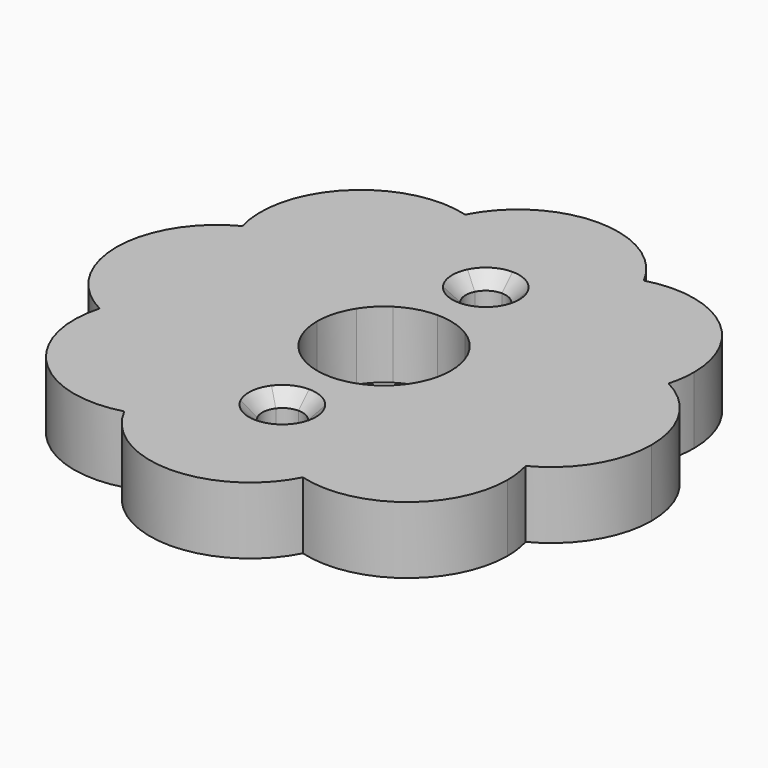
from build123d import *

# Parameters (mm, degrees)
F1_DEPTH = 6.35
F2_SIZE  = 1.27


with BuildPart() as f1:
    # F0 (on Top) → F1 (new body)
    with BuildSketch(Plane.XY):
        with BuildLine():
            Line((9.0862708935, 13.0175), (13.0175, 9.0862708935))
            ThreePointArc((13.0175, 9.0862708935), (11.2253201513, 11.2253201513), (9.0862708935, 13.0175))
        make_face()
        with BuildLine():
            ThreePointArc((20.221779693, 8.4753248493), (16.6798616454, 9.4909337123), (13.0175, 9.0862708935))
            ThreePointArc((13.0175, 9.0862708935), (14.680846164, 6.0405613073), (15.6426389263, 2.7061914978))
            ThreePointArc((15.6426389263, 2.7061914978), (18.5124203716, 5.1302265884), (20.221779693, 8.4753248493))
        make_face()
        with BuildLine():
            ThreePointArc((9.0862708935, 13.0175), (11.2253201513, 11.2253201513), (13.0175, 9.0862708935))
            ThreePointArc((13.0175, 9.0862708935), (16.6798616454, 9.4909337123), (20.221779693, 8.4753248493))
            ThreePointArc((20.221779693, 8.4753248493), (20.4876913926, 9.751427392), (20.5768854467, 11.0518854467))
            ThreePointArc((20.5768854467, 11.0518854467), (16.8044451078, 18.6435705262), (8.4753248493, 20.221779693))
            ThreePointArc((8.4753248493, 20.221779693), (9.2588631643, 18.1108617814), (9.525, 15.875))
            ThreePointArc((9.525, 15.875), (9.4146788384, 14.4295079143), (9.0862708935, 13.0175))
        make_face()
        with BuildLine():
            ThreePointArc((15.6426389263, 2.7061914978), (14.680846164, 6.0405613073), (13.0175, 9.0862708935))
            ThreePointArc((13.0175, 9.0862708935), (9.0369714008, 6.6307608822), (6.7051057537, 2.5765605975))
            ThreePointArc((6.7051057537, 2.5765605975), (11.1900224972, 1.5278871711), (15.6426389263, 2.7061914978))
        make_face()
        with BuildLine():
            ThreePointArc((6.7051057537, 2.5765605975), (9.0369714008, 6.6307608822), (13.0175, 9.0862708935))
            Line((13.0175, 9.0862708935), (9.0862708935, 13.0175))
            ThreePointArc((9.0862708935, 13.0175), (6.6307608822, 9.0369714008), (2.5765605975, 6.7051057537))
            ThreePointArc((2.5765605975, 6.7051057537), (2.9714834378, 6.0087982599), (3.4234793231, 5.3481108183))
            ThreePointArc((3.4234793231, 5.3481108183), (4.4901280605, 4.4901280605), (5.3481108183, 3.4234793231))
            ThreePointArc((5.3481108183, 3.4234793231), (6.0087982599, 2.9714834378), (6.7051057537, 2.5765605975))
        make_face()
        with BuildLine():
            ThreePointArc((2.5765605975, 6.7051057537), (6.6307608822, 9.0369714008), (9.0862708935, 13.0175))
            ThreePointArc((9.0862708935, 13.0175), (6.0405613073, 14.680846164), (2.7061914978, 15.6426389263))
            ThreePointArc((2.7061914978, 15.6426389263), (2.1024733841, 14.3128130347), (1.7091513138, 12.9063244241))
            ThreePointArc((1.7091513138, 12.9063244241), (1.8553919064, 12.4969095665), (1.905, 12.065))
            ThreePointArc((1.905, 12.065), (1.8082177094, 11.465522131), (1.5277047607, 10.9269564313))
            ThreePointArc((1.5277047607, 10.9269564313), (1.8078843831, 8.7553512461), (2.5765605975, 6.7051057537))
        make_face()
        with BuildLine():
            ThreePointArc((2.7061914978, 15.6426389263), (6.0405613073, 14.680846164), (9.0862708935, 13.0175))
            ThreePointArc((9.0862708935, 13.0175), (9.4146788384, 14.4295079143), (9.525, 15.875))
            ThreePointArc((9.525, 15.875), (9.2588631643, 18.1108617814), (8.4753248493, 20.221779693))
            ThreePointArc((8.4753248493, 20.221779693), (5.1302265884, 18.5124203716), (2.7061914978, 15.6426389263))
        make_face()
        with BuildLine():
            ThreePointArc((20.221779693, 8.4753248493), (18.5124203716, 5.1302265884), (15.6426389263, 2.7061914978))
            ThreePointArc((15.6426389263, 2.7061914978), (15.8168030581, 1.3580743804), (15.875, 0))
            ThreePointArc((15.875, 0), (15.8168030581, -1.3580743804), (15.6426389263, -2.7061914978))
            ThreePointArc((15.6426389263, -2.7061914978), (18.5124203716, -5.1302265884), (20.221779693, -8.4753248493))
            ThreePointArc((20.221779693, -8.4753248493), (24.0029979569, -4.9660119021), (25.4, 0))
            ThreePointArc((25.4, 0), (24.0029979569, 4.9660119021), (20.221779693, 8.4753248493))
        make_face()
        with BuildLine():
            ThreePointArc((15.875, 0), (15.8168030581, 1.3580743804), (15.6426389263, 2.7061914978))
            ThreePointArc((15.6426389263, 2.7061914978), (11.1900224972, 1.5278871711), (6.7051057537, 2.5765605975))
            ThreePointArc((6.7051057537, 2.5765605975), (6.4391940541, 1.3004580548), (6.35, 0))
            Line((6.35, 0), (15.875, 0))
        make_face()
        with BuildLine():
            ThreePointArc((6.35, 0), (6.4391940541, 1.3004580548), (6.7051057537, 2.5765605975))
            ThreePointArc((6.7051057537, 2.5765605975), (6.0087982599, 2.9714834378), (5.3481108183, 3.4234793231))
            ThreePointArc((5.3481108183, 3.4234793231), (6.0943828111, 1.783535296), (6.35, 0))
        make_face()
        with BuildLine():
            ThreePointArc((1.7091513138, 12.9063244241), (2.1024733841, 14.3128130347), (2.7061914978, 15.6426389263))
            ThreePointArc((2.7061914978, 15.6426389263), (1.3580743804, 15.8168030581), (0, 15.875))
            Line((0, 15.875), (0, 13.97))
            ThreePointArc((0, 13.97), (1.0065540155, 13.6823663821), (1.7091513138, 12.9063244241))
        make_face()
        with BuildLine():
            ThreePointArc((0, 15.875), (1.3580743804, 15.8168030581), (2.7061914978, 15.6426389263))
            ThreePointArc((2.7061914978, 15.6426389263), (5.1302265884, 18.5124203716), (8.4753248493, 20.221779693))
            ThreePointArc((8.4753248493, 20.221779693), (0, 25.4), (-8.4753248493, 20.221779693))
            ThreePointArc((-8.4753248493, 20.221779693), (-5.1302265884, 18.5124203716), (-2.7061914978, 15.6426389263))
            ThreePointArc((-2.7061914978, 15.6426389263), (-1.3580743804, 15.8168030581), (0, 15.875))
        make_face()
        with BuildLine():
            ThreePointArc((3.4234793231, 5.3481108183), (2.9714834378, 6.0087982599), (2.5765605975, 6.7051057537))
            ThreePointArc((2.5765605975, 6.7051057537), (1.3004580548, 6.4391940541), (0, 6.35))
            ThreePointArc((0, 6.35), (1.783535296, 6.0943828111), (3.4234793231, 5.3481108183))
        make_face()
        with BuildLine():
            ThreePointArc((0, 6.35), (1.3004580548, 6.4391940541), (2.5765605975, 6.7051057537))
            ThreePointArc((2.5765605975, 6.7051057537), (1.8078843831, 8.7553512461), (1.5277047607, 10.9269564313))
            ThreePointArc((1.5277047607, 10.9269564313), (0.8547081378, 10.3625021295), (0, 10.16))
            Line((0, 10.16), (0, 6.35))
        make_face()
        with BuildLine():
            ThreePointArc((15.6426389263, -2.7061914978), (15.8168030581, -1.3580743804), (15.875, 0))
            Line((15.875, 0), (6.35, 0))
            ThreePointArc((6.35, 0), (6.4391940541, -1.3004580548), (6.7051057537, -2.5765605975))
            ThreePointArc((6.7051057537, -2.5765605975), (11.1900224972, -1.5278871711), (15.6426389263, -2.7061914978))
        make_face()
        with BuildLine():
            ThreePointArc((6.7051057537, -2.5765605975), (6.4391940541, -1.3004580548), (6.35, 0))
            ThreePointArc((6.35, 0), (6.0943828111, -1.783535296), (5.3481108183, -3.4234793231))
            ThreePointArc((5.3481108183, -3.4234793231), (6.0087982599, -2.9714834378), (6.7051057537, -2.5765605975))
        make_face()
        with BuildLine():
            Line((0, 13.97), (0, 15.875))
            ThreePointArc((0, 15.875), (-1.3580743804, 15.8168030581), (-2.7061914978, 15.6426389263))
            ThreePointArc((-2.7061914978, 15.6426389263), (-2.1024733841, 14.3128130347), (-1.7091513138, 12.9063244241))
            ThreePointArc((-1.7091513138, 12.9063244241), (-1.0065540155, 13.6823663821), (0, 13.97))
        make_face()
        with BuildLine():
            ThreePointArc((-2.5765605975, 6.7051057537), (-1.3004580548, 6.4391940541), (0, 6.35))
            Line((0, 6.35), (0, 10.16))
            ThreePointArc((0, 10.16), (-0.8547081378, 10.3625021295), (-1.5277047607, 10.9269564313))
            ThreePointArc((-1.5277047607, 10.9269564313), (-1.8078843831, 8.7553512461), (-2.5765605975, 6.7051057537))
        make_face()
        with BuildLine():
            ThreePointArc((-3.4234793231, 5.3481108183), (-1.783535296, 6.0943828111), (0, 6.35))
            ThreePointArc((0, 6.35), (-1.3004580548, 6.4391940541), (-2.5765605975, 6.7051057537))
            ThreePointArc((-2.5765605975, 6.7051057537), (-2.9714834378, 6.0087982599), (-3.4234793231, 5.3481108183))
        make_face()
        with BuildLine():
            ThreePointArc((20.221779693, -8.4753248493), (18.5124203716, -5.1302265884), (15.6426389263, -2.7061914978))
            ThreePointArc((15.6426389263, -2.7061914978), (14.680846164, -6.0405613073), (13.0175, -9.0862708935))
            ThreePointArc((13.0175, -9.0862708935), (16.6798616454, -9.4909337123), (20.221779693, -8.4753248493))
        make_face()
        with BuildLine():
            ThreePointArc((13.0175, -9.0862708935), (14.680846164, -6.0405613073), (15.6426389263, -2.7061914978))
            ThreePointArc((15.6426389263, -2.7061914978), (11.1900224972, -1.5278871711), (6.7051057537, -2.5765605975))
            ThreePointArc((6.7051057537, -2.5765605975), (9.0369714008, -6.6307608822), (13.0175, -9.0862708935))
        make_face()
        with BuildLine():
            ThreePointArc((20.5768854467, -11.0518854467), (20.4876913926, -9.751427392), (20.221779693, -8.4753248493))
            ThreePointArc((20.221779693, -8.4753248493), (16.6798616454, -9.4909337123), (13.0175, -9.0862708935))
            ThreePointArc((13.0175, -9.0862708935), (11.2253201513, -11.2253201513), (9.0862708935, -13.0175))
            ThreePointArc((9.0862708935, -13.0175), (9.4146788384, -14.4295079143), (9.525, -15.875))
            ThreePointArc((9.525, -15.875), (9.2588631643, -18.1108617814), (8.4753248493, -20.221779693))
            ThreePointArc((8.4753248493, -20.221779693), (16.8044451078, -18.6435705262), (20.5768854467, -11.0518854467))
        make_face()
        with BuildLine():
            ThreePointArc((13.0175, -9.0862708935), (9.0369714008, -6.6307608822), (6.7051057537, -2.5765605975))
            ThreePointArc((6.7051057537, -2.5765605975), (6.0087982599, -2.9714834378), (5.3481108183, -3.4234793231))
            ThreePointArc((5.3481108183, -3.4234793231), (4.4901280605, -4.4901280605), (3.4234793231, -5.3481108183))
            ThreePointArc((3.4234793231, -5.3481108183), (2.9714834378, -6.0087982599), (2.5765605975, -6.7051057537))
            ThreePointArc((2.5765605975, -6.7051057537), (6.6307608822, -9.0369714008), (9.0862708935, -13.0175))
            Line((9.0862708935, -13.0175), (13.0175, -9.0862708935))
        make_face()
        with BuildLine():
            ThreePointArc((-1.7091513138, 12.9063244241), (-2.1024733841, 14.3128130347), (-2.7061914978, 15.6426389263))
            ThreePointArc((-2.7061914978, 15.6426389263), (-6.0405613073, 14.680846164), (-9.0862708935, 13.0175))
            ThreePointArc((-9.0862708935, 13.0175), (-6.6307608822, 9.0369714008), (-2.5765605975, 6.7051057537))
            ThreePointArc((-2.5765605975, 6.7051057537), (-1.8078843831, 8.7553512461), (-1.5277047607, 10.9269564313))
            ThreePointArc((-1.5277047607, 10.9269564313), (-1.8970460523, 11.8910998114), (-1.7091513138, 12.9063244241))
        make_face()
        with BuildLine():
            ThreePointArc((-9.0862708935, 13.0175), (-6.0405613073, 14.680846164), (-2.7061914978, 15.6426389263))
            ThreePointArc((-2.7061914978, 15.6426389263), (-5.1302265884, 18.5124203716), (-8.4753248493, 20.221779693))
            ThreePointArc((-8.4753248493, 20.221779693), (-9.4909337123, 16.6798616454), (-9.0862708935, 13.0175))
        make_face()
        with BuildLine():
            ThreePointArc((-9.0862708935, 13.0175), (-9.4909337123, 16.6798616454), (-8.4753248493, 20.221779693))
            ThreePointArc((-8.4753248493, 20.221779693), (-17.7870775376, 17.7870775376), (-20.221779693, 8.4753248493))
            ThreePointArc((-20.221779693, 8.4753248493), (-16.6798616454, 9.4909337123), (-13.0175, 9.0862708935))
            ThreePointArc((-13.0175, 9.0862708935), (-11.2253201513, 11.2253201513), (-9.0862708935, 13.0175))
        make_face()
        with BuildLine():
            ThreePointArc((-3.4234793231, 5.3481108183), (-2.9714834378, 6.0087982599), (-2.5765605975, 6.7051057537))
            ThreePointArc((-2.5765605975, 6.7051057537), (-6.6307608822, 9.0369714008), (-9.0862708935, 13.0175))
            Line((-9.0862708935, 13.0175), (-13.0175, 9.0862708935))
            ThreePointArc((-13.0175, 9.0862708935), (-9.0369714008, 6.6307608822), (-6.7051057537, 2.5765605975))
            ThreePointArc((-6.7051057537, 2.5765605975), (-6.0087982599, 2.9714834378), (-5.3481108183, 3.4234793231))
            ThreePointArc((-5.3481108183, 3.4234793231), (-4.4901280605, 4.4901280605), (-3.4234793231, 5.3481108183))
        make_face()
        with BuildLine():
            ThreePointArc((9.0862708935, -13.0175), (11.2253201513, -11.2253201513), (13.0175, -9.0862708935))
            Line((13.0175, -9.0862708935), (9.0862708935, -13.0175))
        make_face()
        with BuildLine():
            ThreePointArc((2.5765605975, -6.7051057537), (1.3004580548, -6.4391940541), (0, -6.35))
            Line((0, -6.35), (0, -10.16))
            ThreePointArc((0, -10.16), (0.8547081378, -10.3625021295), (1.5277047607, -10.9269564313))
            ThreePointArc((1.5277047607, -10.9269564313), (1.8078843831, -8.7553512461), (2.5765605975, -6.7051057537))
        make_face()
        with BuildLine():
            ThreePointArc((3.4234793231, -5.3481108183), (1.783535296, -6.0943828111), (0, -6.35))
            ThreePointArc((0, -6.35), (1.3004580548, -6.4391940541), (2.5765605975, -6.7051057537))
            ThreePointArc((2.5765605975, -6.7051057537), (2.9714834378, -6.0087982599), (3.4234793231, -5.3481108183))
        make_face()
        with BuildLine():
            Line((0, -10.16), (0, -6.35))
            ThreePointArc((0, -6.35), (-1.3004580548, -6.4391940541), (-2.5765605975, -6.7051057537))
            ThreePointArc((-2.5765605975, -6.7051057537), (-1.8078843831, -8.7553512461), (-1.5277047607, -10.9269564313))
            ThreePointArc((-1.5277047607, -10.9269564313), (-0.8547081378, -10.3625021295), (0, -10.16))
        make_face()
        with BuildLine():
            ThreePointArc((-2.5765605975, -6.7051057537), (-1.3004580548, -6.4391940541), (0, -6.35))
            ThreePointArc((0, -6.35), (-1.783535296, -6.0943828111), (-3.4234793231, -5.3481108183))
            ThreePointArc((-3.4234793231, -5.3481108183), (-2.9714834378, -6.0087982599), (-2.5765605975, -6.7051057537))
        make_face()
        with BuildLine():
            ThreePointArc((-6.7051057537, -2.5765605975), (-6.4391940541, -1.3004580548), (-6.35, 0))
            Line((-6.35, 0), (-15.875, 0))
            ThreePointArc((-15.875, 0), (-15.8168030581, -1.3580743804), (-15.6426389263, -2.7061914978))
            ThreePointArc((-15.6426389263, -2.7061914978), (-11.1900224972, -1.5278871711), (-6.7051057537, -2.5765605975))
        make_face()
        with BuildLine():
            Line((-15.875, 0), (-6.35, 0))
            ThreePointArc((-6.35, 0), (-6.4391940541, 1.3004580548), (-6.7051057537, 2.5765605975))
            ThreePointArc((-6.7051057537, 2.5765605975), (-11.1900224972, 1.5278871711), (-15.6426389263, 2.7061914978))
            ThreePointArc((-15.6426389263, 2.7061914978), (-15.8168030581, 1.3580743804), (-15.875, 0))
        make_face()
        with BuildLine():
            ThreePointArc((-5.3481108183, -3.4234793231), (-6.0943828111, -1.783535296), (-6.35, 0))
            ThreePointArc((-6.35, 0), (-6.4391940541, -1.3004580548), (-6.7051057537, -2.5765605975))
            ThreePointArc((-6.7051057537, -2.5765605975), (-6.0087982599, -2.9714834378), (-5.3481108183, -3.4234793231))
        make_face()
        with BuildLine():
            ThreePointArc((-6.7051057537, 2.5765605975), (-6.4391940541, 1.3004580548), (-6.35, 0))
            ThreePointArc((-6.35, 0), (-6.0943828111, 1.783535296), (-5.3481108183, 3.4234793231))
            ThreePointArc((-5.3481108183, 3.4234793231), (-6.0087982599, 2.9714834378), (-6.7051057537, 2.5765605975))
        make_face()
        with BuildLine():
            Line((-13.0175, 9.0862708935), (-9.0862708935, 13.0175))
            ThreePointArc((-9.0862708935, 13.0175), (-11.2253201513, 11.2253201513), (-13.0175, 9.0862708935))
        make_face()
        with BuildLine():
            ThreePointArc((-15.6426389263, 2.7061914978), (-18.5124203716, 5.1302265884), (-20.221779693, 8.4753248493))
            ThreePointArc((-20.221779693, 8.4753248493), (-25.4, 0), (-20.221779693, -8.4753248493))
            ThreePointArc((-20.221779693, -8.4753248493), (-18.5124203716, -5.1302265884), (-15.6426389263, -2.7061914978))
            ThreePointArc((-15.6426389263, -2.7061914978), (-15.8168030581, -1.3580743804), (-15.875, 0))
            ThreePointArc((-15.875, 0), (-15.8168030581, 1.3580743804), (-15.6426389263, 2.7061914978))
        make_face()
        with BuildLine():
            ThreePointArc((-13.0175, 9.0862708935), (-16.6798616454, 9.4909337123), (-20.221779693, 8.4753248493))
            ThreePointArc((-20.221779693, 8.4753248493), (-18.5124203716, 5.1302265884), (-15.6426389263, 2.7061914978))
            ThreePointArc((-15.6426389263, 2.7061914978), (-14.680846164, 6.0405613073), (-13.0175, 9.0862708935))
        make_face()
        with BuildLine():
            ThreePointArc((9.525, -15.875), (9.4146788384, -14.4295079143), (9.0862708935, -13.0175))
            ThreePointArc((9.0862708935, -13.0175), (6.0405613073, -14.680846164), (2.7061914978, -15.6426389263))
            ThreePointArc((2.7061914978, -15.6426389263), (5.1302265884, -18.5124203716), (8.4753248493, -20.221779693))
            ThreePointArc((8.4753248493, -20.221779693), (9.2588631643, -18.1108617814), (9.525, -15.875))
        make_face()
        with BuildLine():
            ThreePointArc((2.7061914978, -15.6426389263), (6.0405613073, -14.680846164), (9.0862708935, -13.0175))
            ThreePointArc((9.0862708935, -13.0175), (6.6307608822, -9.0369714008), (2.5765605975, -6.7051057537))
            ThreePointArc((2.5765605975, -6.7051057537), (1.8078843831, -8.7553512461), (1.5277047607, -10.9269564313))
            ThreePointArc((1.5277047607, -10.9269564313), (1.8082177094, -11.465522131), (1.905, -12.065))
            ThreePointArc((1.905, -12.065), (1.8553919064, -12.4969095665), (1.7091513138, -12.9063244241))
            ThreePointArc((1.7091513138, -12.9063244241), (2.1024733841, -14.3128130347), (2.7061914978, -15.6426389263))
        make_face()
        with BuildLine():
            ThreePointArc((-8.4753248493, -20.221779693), (0, -25.4), (8.4753248493, -20.221779693))
            ThreePointArc((8.4753248493, -20.221779693), (5.1302265884, -18.5124203716), (2.7061914978, -15.6426389263))
            ThreePointArc((2.7061914978, -15.6426389263), (1.3580743804, -15.8168030581), (0, -15.875))
            ThreePointArc((0, -15.875), (-1.3580743804, -15.8168030581), (-2.7061914978, -15.6426389263))
            ThreePointArc((-2.7061914978, -15.6426389263), (-5.1302265884, -18.5124203716), (-8.4753248493, -20.221779693))
        make_face()
        with BuildLine():
            ThreePointArc((-1.5277047607, -10.9269564313), (-1.8078843831, -8.7553512461), (-2.5765605975, -6.7051057537))
            ThreePointArc((-2.5765605975, -6.7051057537), (-6.6307608822, -9.0369714008), (-9.0862708935, -13.0175))
            ThreePointArc((-9.0862708935, -13.0175), (-6.0405613073, -14.680846164), (-2.7061914978, -15.6426389263))
            ThreePointArc((-2.7061914978, -15.6426389263), (-2.1024733841, -14.3128130347), (-1.7091513138, -12.9063244241))
            ThreePointArc((-1.7091513138, -12.9063244241), (-1.8970460523, -11.8910998114), (-1.5277047607, -10.9269564313))
        make_face()
        with BuildLine():
            ThreePointArc((-9.0862708935, -13.0175), (-6.6307608822, -9.0369714008), (-2.5765605975, -6.7051057537))
            ThreePointArc((-2.5765605975, -6.7051057537), (-2.9714834378, -6.0087982599), (-3.4234793231, -5.3481108183))
            ThreePointArc((-3.4234793231, -5.3481108183), (-4.4901280605, -4.4901280605), (-5.3481108183, -3.4234793231))
            ThreePointArc((-5.3481108183, -3.4234793231), (-6.0087982599, -2.9714834378), (-6.7051057537, -2.5765605975))
            ThreePointArc((-6.7051057537, -2.5765605975), (-9.0369714008, -6.6307608822), (-13.0175, -9.0862708935))
            Line((-13.0175, -9.0862708935), (-9.0862708935, -13.0175))
        make_face()
        with BuildLine():
            ThreePointArc((-15.6426389263, 2.7061914978), (-11.1900224972, 1.5278871711), (-6.7051057537, 2.5765605975))
            ThreePointArc((-6.7051057537, 2.5765605975), (-9.0369714008, 6.6307608822), (-13.0175, 9.0862708935))
            ThreePointArc((-13.0175, 9.0862708935), (-14.680846164, 6.0405613073), (-15.6426389263, 2.7061914978))
        make_face()
        with BuildLine():
            ThreePointArc((-13.0175, -9.0862708935), (-9.0369714008, -6.6307608822), (-6.7051057537, -2.5765605975))
            ThreePointArc((-6.7051057537, -2.5765605975), (-11.1900224972, -1.5278871711), (-15.6426389263, -2.7061914978))
            ThreePointArc((-15.6426389263, -2.7061914978), (-14.680846164, -6.0405613073), (-13.0175, -9.0862708935))
        make_face()
        with BuildLine():
            ThreePointArc((-15.6426389263, -2.7061914978), (-18.5124203716, -5.1302265884), (-20.221779693, -8.4753248493))
            ThreePointArc((-20.221779693, -8.4753248493), (-16.6798616454, -9.4909337123), (-13.0175, -9.0862708935))
            ThreePointArc((-13.0175, -9.0862708935), (-14.680846164, -6.0405613073), (-15.6426389263, -2.7061914978))
        make_face()
        with BuildLine():
            ThreePointArc((-13.0175, -9.0862708935), (-16.6798616454, -9.4909337123), (-20.221779693, -8.4753248493))
            ThreePointArc((-20.221779693, -8.4753248493), (-17.7870775376, -17.7870775376), (-8.4753248493, -20.221779693))
            ThreePointArc((-8.4753248493, -20.221779693), (-9.4909337123, -16.6798616454), (-9.0862708935, -13.0175))
            ThreePointArc((-9.0862708935, -13.0175), (-11.2253201513, -11.2253201513), (-13.0175, -9.0862708935))
        make_face()
        with BuildLine():
            ThreePointArc((0, -15.875), (1.3580743804, -15.8168030581), (2.7061914978, -15.6426389263))
            ThreePointArc((2.7061914978, -15.6426389263), (2.1024733841, -14.3128130347), (1.7091513138, -12.9063244241))
            ThreePointArc((1.7091513138, -12.9063244241), (1.0065540155, -13.6823663821), (0, -13.97))
            Line((0, -13.97), (0, -15.875))
        make_face()
        with BuildLine():
            ThreePointArc((-9.0862708935, -13.0175), (-9.4909337123, -16.6798616454), (-8.4753248493, -20.221779693))
            ThreePointArc((-8.4753248493, -20.221779693), (-5.1302265884, -18.5124203716), (-2.7061914978, -15.6426389263))
            ThreePointArc((-2.7061914978, -15.6426389263), (-6.0405613073, -14.680846164), (-9.0862708935, -13.0175))
        make_face()
        with BuildLine():
            Line((0, -15.875), (0, -13.97))
            ThreePointArc((0, -13.97), (-1.0065540155, -13.6823663821), (-1.7091513138, -12.9063244241))
            ThreePointArc((-1.7091513138, -12.9063244241), (-2.1024733841, -14.3128130347), (-2.7061914978, -15.6426389263))
            ThreePointArc((-2.7061914978, -15.6426389263), (-1.3580743804, -15.8168030581), (0, -15.875))
        make_face()
        with BuildLine():
            ThreePointArc((-13.0175, -9.0862708935), (-11.2253201513, -11.2253201513), (-9.0862708935, -13.0175))
            Line((-9.0862708935, -13.0175), (-13.0175, -9.0862708935))
        make_face()
    extrude(amount=F1_DEPTH)

    # F2
    f2_edges = [f1.edges().sort_by_distance(p)[0] for p in [
        (-1.709151, -11.223676, 6.35),
        (-1.527705, 13.203044, 6.35),
    ]]
    chamfer(f2_edges, length=F2_SIZE)


solid = f1.part
